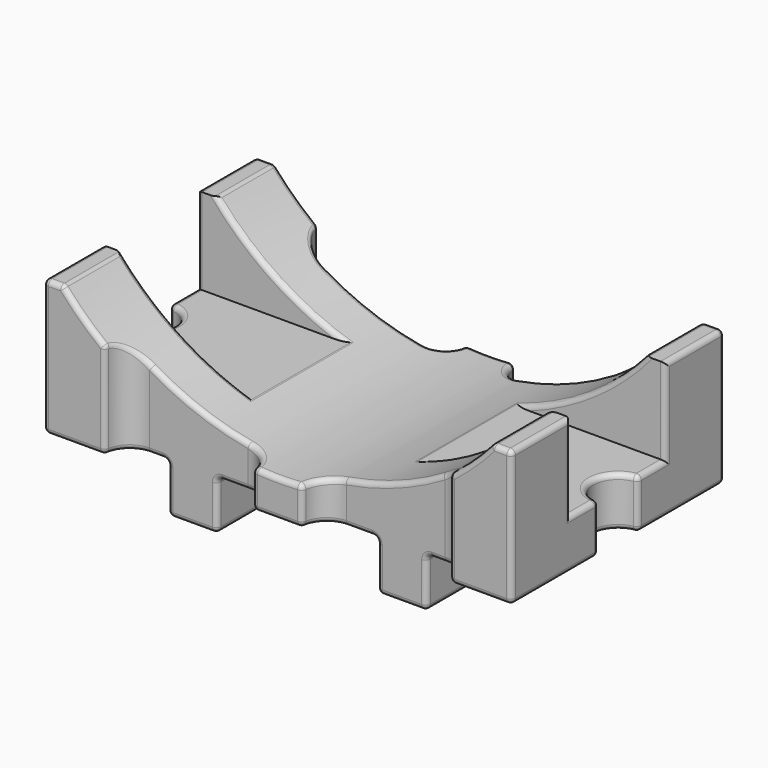
from build123d import *

# Parameters (mm, degrees)
F1_START = 2
F0_W     = 19
F0_H     = 10.8
F1_DEPTH = 5.5
F2_W     = 2
F2_H     = 10
F3_DEPTH = 2
F5_START = 4
F4_W     = 26
F4_H     = 4.8
F5_DEPTH = 6
F6_R     = 11.5
F7_DEPTH = 12.5
F8_R     = 1
F9_DEPTH = 10
F10_F1_R = 0.2
F10_F2_R = 0.2


with BuildPart() as f1:
    # F0 (on Top) → F1 (new body)
    with BuildSketch(Plane.XY.offset(F1_START)):
        Rectangle(F0_W, F0_H)
    extrude(amount=F1_DEPTH)

    # F2 (on Top) → F3 (join)
    with BuildSketch(Plane.XY):
        with Locations((4.25, -0.0206499083)):
            Rectangle(F2_W, F2_H)
        with Locations((-4.25, -0.0212505543)):
            Rectangle(F2_W, F2_H)
    extrude(amount=F3_DEPTH)

    # F4 (on Top) → F5 (cut)
    with BuildSketch(Plane.XY.offset(F5_START)):
        Rectangle(F4_W, F4_H)
    extrude(amount=F5_DEPTH, mode=Mode.SUBTRACT)

    # F6 (on Front) → F7 (cut, symmetric)
    with BuildSketch(Plane.XZ):
        with Locations((0, 15)):
            Circle(F6_R)
    extrude(amount=F7_DEPTH, both=True, mode=Mode.SUBTRACT)

    # F8 (on Top) → F9 (cut)
    with BuildSketch(Plane.XY):
        with Locations((-9.5, 0)):
            Circle(F8_R)
        with BuildLine():
            Line((-1, 6.4), (-7, 6.4))
            Line((-7, 6.4), (-7, 5.4))
            ThreePointArc((-7, 5.4), (-6.7071067812, 4.6928932188), (-6, 4.4))
            Line((-6, 4.4), (-2, 4.4))
            ThreePointArc((-2, 4.4), (-1.2928932188, 4.6928932188), (-1, 5.4))
            Line((-1, 5.4), (-1, 6.4))
        make_face()
        with BuildLine():
            ThreePointArc((1, 5.4), (1.2928932188, 4.6928932188), (2, 4.4))
            Line((2, 4.4), (6, 4.4))
            ThreePointArc((6, 4.4), (6.7071067812, 4.6928932188), (7, 5.4))
            Line((7, 5.4), (7, 6.4))
            Line((7, 6.4), (1, 6.4))
            Line((1, 6.4), (1, 5.4))
        make_face()
        with Locations((9.5010781661, 0)):
            Circle(F8_R)
        with BuildLine():
            Line((7, -6.4), (7, -5.4))
            ThreePointArc((7, -5.4), (6.7071067812, -4.6928932188), (6, -4.4))
            Line((6, -4.4), (2, -4.4))
            ThreePointArc((2, -4.4), (1.2928932188, -4.6928932188), (1, -5.4))
            Line((1, -5.4), (1, -6.4))
            Line((1, -6.4), (7, -6.4))
        make_face()
        with BuildLine():
            ThreePointArc((-1, -5.4), (-1.2928932188, -4.6928932188), (-2, -4.4))
            Line((-2, -4.4), (-6, -4.4))
            ThreePointArc((-6, -4.4), (-6.7071067812, -4.6928932188), (-7, -5.4))
            Line((-7, -5.4), (-7, -6.4))
            Line((-7, -6.4), (-1, -6.4))
            Line((-1, -6.4), (-1, -5.4))
        make_face()
    extrude(amount=F9_DEPTH, mode=Mode.SUBTRACT)

    # F10: fillet of radius 0.2 on 94 edges, made by hand

    # F10_f1
    f10_f1_edges = [f1.edges().sort_by_distance(p)[0] for p in [
        (-3.25, 0, 2),
        (5.25, 0, 2),
        (3.25, 0, 2),
        (-5.25, 0, 2),
    ]]
    fillet(f10_f1_edges, radius=F10_F1_R)

    # F10_f2
    f10_f2_edges = [f1.edges().sort_by_distance(p)[0] for p in [
        (-9.5, -3.9, 7.5),
        (-7.9007438493, -5.4, 6.6436702657),
        (-6.7121815661, -4.6980047363, 5.6620870366),
        (-4.0710050008, -4.4, 4.244679536),
        (-1.2591693657, -4.7283081163, 3.5691429685),
        (0, -5.4, 3.5),
        (1.262028341, -4.7251682939, 3.5694582627),
        (4.0710050008, -4.4, 4.244679536),
        (6.7121817502, -4.6980049232, 5.662087169),
        (7.9007438493, -5.4, 6.6436702657),
        (8.7177978871, -3.9, 7.5),
        (6.284519991, -2.4, 5.3690702171),
        (3.3541019662, 0, 4),
        (6.284519991, 2.4, 5.3690702171),
        (8.7177978871, 3.9, 7.5),
        (7.9007438493, 5.4, 6.6436702657),
        (6.7121815661, 4.6980047363, 5.6620870366),
        (4.0710050008, 4.4, 4.244679536),
        (1.2591693657, 4.7283081163, 3.5691429685),
        (0, 5.4, 3.5),
        (-1.2620283411, 4.7251682938, 3.5694582627),
        (-4.0710050008, 4.4, 4.244679536),
        (-6.7121822556, 4.698005436, 5.6620875323),
        (-7.9007438493, 5.4, 6.6436702657),
        (-8.7177978871, 3.9, 7.5),
        (-6.284519991, 2.4, 5.3690702171),
        (-3.3541019662, 0, 4),
        (-6.284519991, -2.4, 5.3690702171),
        (-8.7177978871, -3.9, 7.5),
        (9.5, -3.1999997094, 2),
        (9.5, -0.9999994188, 3),
        (9.5, -1.6999997094, 4),
        (9.5, -2.4, 5.75),
        (9.5, -3.9, 7.5),
        (9.5, -5.4, 4.75),
        (9.5, 3.1999997094, 2),
        (9.5, 5.4, 4.75),
        (9.5, 3.9, 7.5),
        (9.5, 2.4, 5.75),
        (9.5, 1.6999997094, 4),
        (9.5, 0.9999994188, 3),
        (8.25, -5.4, 2),
        (9.1088989435, -5.4, 7.5),
        (7, -5.4, 3.9379281023),
        (0, -5.4, 2),
        (1, -5.4, 2.7717803813),
        (-1, -5.4, 2.7717803813),
        (-8.25, -5.4, 2),
        (-7, -5.4, 3.9379281023),
        (-9.1088989435, -5.4, 7.5),
        (-9.5, -5.4, 4.75),
        (-9.5, -3.2, 2),
        (-9.5, -2.4, 5.75),
        (-9.5, -1.7, 4),
        (-9.5, -1, 3),
        (-9.5, 3.2, 2),
        (-9.5, 1, 3),
        (-9.5, 1.7, 4),
        (-9.5, 2.4, 5.75),
        (-9.5, 3.9, 7.5),
        (-9.5, 5.4, 4.75),
        (-8.25, 5.4, 2),
        (-9.1088989435, 5.4, 7.5),
        (-7, 5.4, 3.9379281023),
        (0, 5.4, 2),
        (-1, 5.4, 2.7717803813),
        (1, 5.4, 2.7717803813),
        (8.25, 5.4, 2),
        (7, 5.4, 3.9379281023),
        (9.1088989435, 5.4, 7.5),
        (-3.25, 0, 0),
        (-3.25, 4.4, 0.9),
        (-3.25, -4.4, 0.9),
        (5.25, 0, 0),
        (5.25, 4.4, 0.9),
        (5.25, -4.4, 0.9),
        (3.25, 0, 0),
        (3.25, -4.4, 0.9),
        (3.25, 4.4, 0.9),
        (-5.25, 0, 0),
        (-5.25, -4.4, 0.9),
        (-5.25, 4.4, 0.9),
        (-4.25, -4.4, 0),
        (4.25, -4.4, 0),
        (-4.25, 4.4, 0),
        (4.25, 4.4, 0),
        (8.5010781661, 0, 2),
        (-8.5, 0, 2),
        (-8.5, 0, 4),
        (8.5010781661, 0, 4),
        (-5.3085786438, 4.4, 1.9414213562),
        (-5.3085786438, -4.4, 1.9414213562),
        (3.1914213562, 4.4, 1.9414213562),
        (3.1914213562, -4.4, 1.9414213562),
        (5.3085786438, -4.4, 1.9414213562),
        (5.3085786438, 4.4, 1.9414213562),
        (-3.1914213562, -4.4, 1.9414213562),
        (-3.1914213562, 4.4, 1.9414213562),
    ]]
    fillet(f10_f2_edges, radius=F10_F2_R)


solid = f1.part
